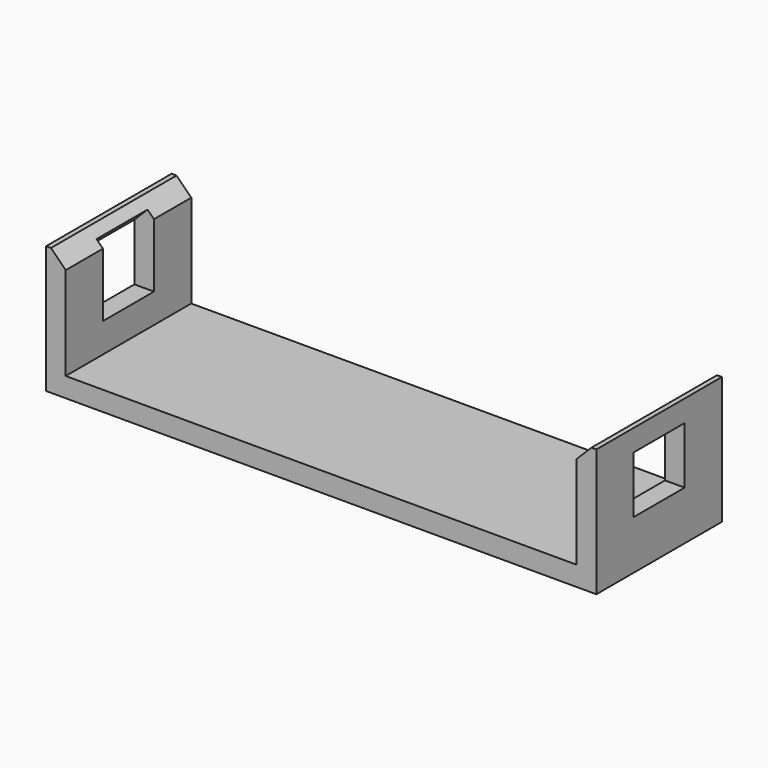
from build123d import *

# Parameters (mm, degrees)
F0_W        = 52.1
F0_H        = 16
F1_DEPTH    = 5
F2_W        = 2
F2_H        = 16
F3_DEPTH    = 16
F4_W        = 6.5
F4_H        = 5.3
F5_DEPTH    = 195
F6_SIZE     = 1.5
F7_T1_DEPTH = 6.5
F8_DEPTH    = 3


# Not quite as in the source:
# - a fillet or chamfer that OpenCascade refuses, or shapes differently, is made with other operations: its cross-section is extruded or revolved along the edge and cut away or added


with BuildPart() as f1:
    # F0 (on Top) → F1 (new body)
    with BuildSketch(Plane.XY):
        with Locations((26.05, -8)):
            Rectangle(F0_W, F0_H)
    extrude(amount=F1_DEPTH)

    # F2 (on Top) → F3 (join)
    with BuildSketch(Plane.XY):
        with Locations((-1, -8)):
            Rectangle(F2_W, F2_H)
        with Locations((53.1, -8)):
            Rectangle(F2_W, F2_H)
    extrude(amount=F3_DEPTH)

    # F4 (on face) → F5 (cut, symmetric)
    with BuildSketch(Plane(origin=(52.1, 0, 0), x_dir=(0, -1, 0), z_dir=(-1, 0, 0))):
        with Locations((8, 10.65)):
            Rectangle(F4_W, F4_H)
    extrude(amount=F5_DEPTH, both=True, mode=Mode.SUBTRACT)

    # F6
    f6_edges = [f1.edges().sort_by_distance(p)[0] for p in [
        (52.1, -8, 16),
        (0, -8, 16),
    ]]
    chamfer(f6_edges, length=F6_SIZE)

    # F7: chamfer of 2.5 on 2 edges, made by hand

    # F7_s2 → F7_t1 (cut)
    with BuildSketch(Plane.XZ.offset(4.75)):
        Polygon((52.1, 15.8), (54.6, 13.3), (52.1, 13.3), align=None)
        Polygon((0, 15.8), (-2.5, 13.3), (0, 13.3), align=None)
    extrude(amount=F7_T1_DEPTH, mode=Mode.SUBTRACT)

    # F8 (cut): a face of the model
    f8_faces = [f1.faces().sort_by_distance(p)[0] for p in [
        (26.05, -8, 0),
    ]]
    extrude(f8_faces, amount=-F8_DEPTH, mode=Mode.SUBTRACT)


solid = f1.part
